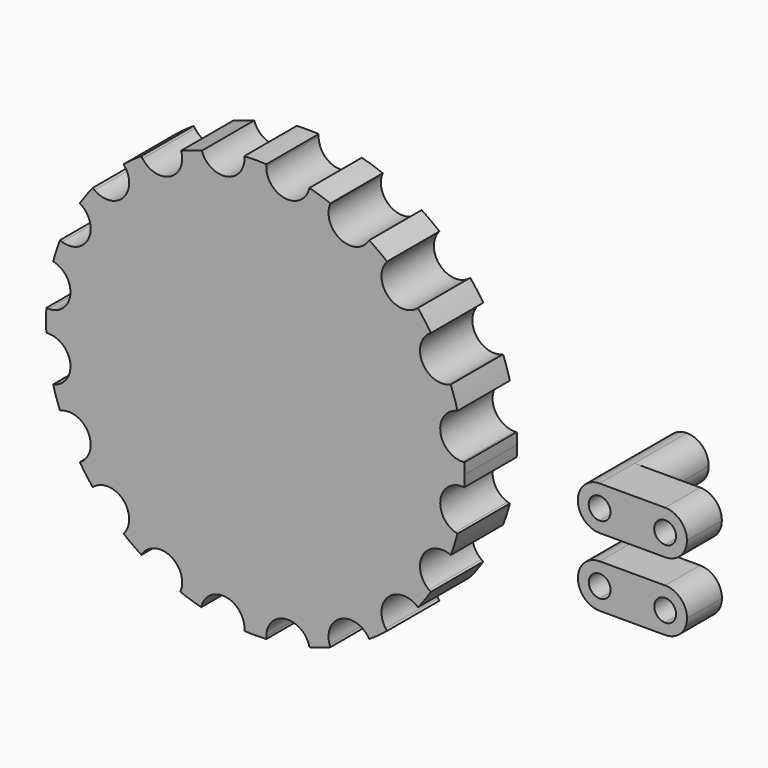
from build123d import *

# Parameters (mm, degrees)
F1_DEPTH = 15
F2_DEPTH = 10
F3_DEPTH = 15
F4_DEPTH = 10


with BuildPart() as f1:
    # F0 (on Front) → F1 (new body)
    with BuildSketch(Plane.XZ):
        with BuildLine():
            Line((47.3531363601, -2.5), (47.3531363601, 2.5))
            ThreePointArc((47.3531363601, 2.5), (42.4146946571, 6.7178276748), (45.8080513882, 12.2552825815))
            Line((45.8080513882, 12.2552825815), (44.2629664163, 17.010565163))
            ThreePointArc((44.2629664163, 17.010565163), (38.2628488235, 19.4958952457), (39.778955183, 25.8109327163))
            Line((39.778955183, 25.8109327163), (36.8400289215, 29.8560176882))
            ThreePointArc((36.8400289215, 29.8560176882), (30.3655687541, 30.3655687541), (29.8560176882, 36.8400289215))
            Line((29.8560176882, 36.8400289215), (25.8109327163, 39.778955183))
            ThreePointArc((25.8109327163, 39.778955183), (19.4958952457, 38.2628488235), (17.010565163, 44.2629664163))
            Line((17.010565163, 44.2629664163), (12.2552825815, 45.8080513882))
            ThreePointArc((12.2552825815, 45.8080513882), (6.7178276748, 42.4146946571), (2.5, 47.3531363601))
            Line((2.5, 47.3531363601), (-2.5, 47.3531363601))
            ThreePointArc((-2.5, 47.3531363601), (-6.7178276748, 42.4146946571), (-12.2552825815, 45.8080513882))
            Line((-12.2552825815, 45.8080513882), (-17.010565163, 44.2629664163))
            ThreePointArc((-17.010565163, 44.2629664163), (-16.8274060415, 43.5000537696), (-16.7658477444, 42.7178814444))
            ThreePointArc((-16.7658477444, 42.7178814444), (-20.2207627726, 37.962598863), (-25.8109327163, 39.778955183))
            Line((-25.8109327163, 39.778955183), (-29.8560176882, 36.8400289215))
            ThreePointArc((-29.8560176882, 36.8400289215), (-29.1458200786, 35.4461876319), (-28.9011026601, 33.9011026601))
            ThreePointArc((-28.9011026601, 33.9011026601), (-31.6311501614, 29.4460700391), (-36.8400289215, 29.8560176882))
            Line((-36.8400289215, 29.8560176882), (-39.778955183, 25.8109327163))
            ThreePointArc((-39.778955183, 25.8109327163), (-38.2628488235, 24.0358002431), (-37.7178814444, 21.7658477444))
            ThreePointArc((-37.7178814444, 21.7658477444), (-39.778955183, 17.7207627726), (-44.2629664163, 17.010565163))
            Line((-44.2629664163, 17.010565163), (-45.8080513882, 12.2552825815))
            ThreePointArc((-45.8080513882, 12.2552825815), (-43.3080513882, 10.4389262615), (-42.3531363601, 7.5))
            ThreePointArc((-42.3531363601, 7.5), (-43.8176024541, 3.9644660941), (-47.3531363601, 2.5))
            Line((-47.3531363601, 2.5), (-47.3531363601, -2.5))
            ThreePointArc((-47.3531363601, -2.5), (-43.8176024541, -3.9644660941), (-42.3531363601, -7.5))
            ThreePointArc((-42.3531363601, -7.5), (-43.3080513882, -10.4389262615), (-45.8080513882, -12.2552825815))
            Line((-45.8080513882, -12.2552825815), (-44.2629664163, -17.010565163))
            ThreePointArc((-44.2629664163, -17.010565163), (-39.778955183, -17.7207627726), (-37.7178814444, -21.7658477444))
            ThreePointArc((-37.7178814444, -21.7658477444), (-38.2628488235, -24.0358002431), (-39.778955183, -25.8109327163))
            Line((-39.778955183, -25.8109327163), (-36.8400289215, -29.8560176882))
            ThreePointArc((-36.8400289215, -29.8560176882), (-31.6311501614, -29.4460700391), (-28.9011026601, -33.9011026601))
            ThreePointArc((-28.9011026601, -33.9011026601), (-29.1458200786, -35.4461876319), (-29.8560176882, -36.8400289215))
            Line((-29.8560176882, -36.8400289215), (-25.8109327163, -39.778955183))
            ThreePointArc((-25.8109327163, -39.778955183), (-20.2207627726, -37.962598863), (-16.7658477444, -42.7178814444))
            ThreePointArc((-16.7658477444, -42.7178814444), (-16.8274060415, -43.5000537696), (-17.010565163, -44.2629664163))
            Line((-17.010565163, -44.2629664163), (-12.2552825815, -45.8080513882))
            ThreePointArc((-12.2552825815, -45.8080513882), (-6.7178276748, -42.4146946571), (-2.5, -47.3531363601))
            Line((-2.5, -47.3531363601), (2.5, -47.3531363601))
            ThreePointArc((2.5, -47.3531363601), (6.7178276748, -42.4146946571), (12.2552825815, -45.8080513882))
            Line((12.2552825815, -45.8080513882), (17.010565163, -44.2629664163))
            ThreePointArc((17.010565163, -44.2629664163), (19.4958952457, -38.2628488235), (25.8109327163, -39.778955183))
            Line((25.8109327163, -39.778955183), (29.8560176882, -36.8400289215))
            ThreePointArc((29.8560176882, -36.8400289215), (30.3655687541, -30.3655687541), (36.8400289215, -29.8560176882))
            Line((36.8400289215, -29.8560176882), (39.778955183, -25.8109327163))
            ThreePointArc((39.778955183, -25.8109327163), (38.2628488235, -19.4958952457), (44.2629664163, -17.010565163))
            Line((44.2629664163, -17.010565163), (45.8080513882, -12.2552825815))
            ThreePointArc((45.8080513882, -12.2552825815), (42.4146946571, -6.7178276748), (47.3531363601, -2.5))
        make_face()
        with BuildLine():
            Line((44.2629664163, 17.010565163), (45.8080513882, 12.2552825815))
            ThreePointArc((45.8080513882, 12.2552825815), (46.0595033261, 12.3297529516), (46.3145139922, 12.3909368813))
            ThreePointArc((46.3145139922, 12.3909368813), (45.5968821856, 14.8153251089), (44.7524388669, 17.1985097785))
            ThreePointArc((44.7524388669, 17.1985097785), (44.5101678926, 17.0981171087), (44.2629664163, 17.010565163))
        make_face()
        with BuildLine():
            ThreePointArc((47.8767304039, 2.5274906458), (47.6152939741, 2.5068773913), (47.3531363601, 2.5))
            Line((47.3531363601, 2.5), (47.3531363601, -2.5))
            ThreePointArc((47.3531363601, -2.5), (47.6152939741, -2.5068773913), (47.8767304039, -2.5274906458))
            ThreePointArc((47.8767304039, -2.5274906458), (47.9267290738, -1.2641848844), (47.9433991612, 0))
            ThreePointArc((47.9433991612, 0), (47.9267290738, 1.2641848844), (47.8767304039, 2.5274906458))
        make_face()
        with BuildLine():
            Line((36.8400289215, 29.8560176882), (39.778955183, 25.8109327163))
            ThreePointArc((39.778955183, 25.8109327163), (39.9950875771, 25.9594611692), (40.2187102588, 26.0964531738))
            ThreePointArc((40.2187102588, 26.0964531738), (38.7870246896, 28.1804229718), (37.247466805, 30.186018945))
            ThreePointArc((37.247466805, 30.186018945), (37.0480764573, 30.0156739939), (36.8400289215, 29.8560176882))
        make_face()
        with BuildLine():
            Line((25.8109327163, 39.778955183), (29.8560176882, 36.8400289215))
            ThreePointArc((29.8560176882, 36.8400289215), (30.0156739939, 37.0480764573), (30.186018945, 37.247466805))
            ThreePointArc((30.186018945, 37.247466805), (28.1804229718, 38.7870246896), (26.0964531738, 40.2187102588))
            ThreePointArc((26.0964531738, 40.2187102588), (25.9594611692, 39.9950875771), (25.8109327163, 39.778955183))
        make_face()
        with BuildLine():
            Line((12.2552825815, 45.8080513882), (17.010565163, 44.2629664163))
            ThreePointArc((17.010565163, 44.2629664163), (17.0981171087, 44.5101678926), (17.1985097785, 44.7524388669))
            ThreePointArc((17.1985097785, 44.7524388669), (14.8153251089, 45.5968821856), (12.3909368813, 46.3145139922))
            ThreePointArc((12.3909368813, 46.3145139922), (12.3297529516, 46.0595033261), (12.2552825815, 45.8080513882))
        make_face()
        with BuildLine():
            Line((-2.5, 47.3531363601), (2.5, 47.3531363601))
            ThreePointArc((2.5, 47.3531363601), (2.5068773913, 47.6152939741), (2.5274906458, 47.8767304039))
            ThreePointArc((2.5274906458, 47.8767304039), (0, 47.9433991612), (-2.5274906458, 47.8767304039))
            ThreePointArc((-2.5274906458, 47.8767304039), (-2.5068773913, 47.6152939741), (-2.5, 47.3531363601))
        make_face()
        with BuildLine():
            ThreePointArc((-25.8109327163, 39.778955183), (-25.9594611692, 39.9950875771), (-26.0964531738, 40.2187102588))
            ThreePointArc((-26.0964531738, 40.2187102588), (-28.1804229718, 38.7870246896), (-30.186018945, 37.247466805))
            ThreePointArc((-30.186018945, 37.247466805), (-30.0156739939, 37.0480764573), (-29.8560176882, 36.8400289215))
            Line((-29.8560176882, 36.8400289215), (-25.8109327163, 39.778955183))
        make_face()
        with BuildLine():
            ThreePointArc((-36.8400289215, 29.8560176882), (-37.0480764573, 30.0156739939), (-37.247466805, 30.186018945))
            ThreePointArc((-37.247466805, 30.186018945), (-38.7870246896, 28.1804229718), (-40.2187102588, 26.0964531738))
            ThreePointArc((-40.2187102588, 26.0964531738), (-39.9950875771, 25.9594611692), (-39.778955183, 25.8109327163))
            Line((-39.778955183, 25.8109327163), (-36.8400289215, 29.8560176882))
        make_face()
        with BuildLine():
            ThreePointArc((-44.2629664163, 17.010565163), (-44.5101678926, 17.0981171087), (-44.7524388669, 17.1985097785))
            ThreePointArc((-44.7524388669, 17.1985097785), (-45.5968821856, 14.8153251089), (-46.3145139922, 12.3909368813))
            ThreePointArc((-46.3145139922, 12.3909368813), (-46.0595033261, 12.3297529516), (-45.8080513882, 12.2552825815))
            Line((-45.8080513882, 12.2552825815), (-44.2629664163, 17.010565163))
        make_face()
        with BuildLine():
            ThreePointArc((-47.3531363601, 2.5), (-47.6152939741, 2.5068773913), (-47.8767304039, 2.5274906458))
            ThreePointArc((-47.8767304039, 2.5274906458), (-47.9433991612, 0), (-47.8767304039, -2.5274906458))
            ThreePointArc((-47.8767304039, -2.5274906458), (-47.6152939741, -2.5068773913), (-47.3531363601, -2.5))
            Line((-47.3531363601, -2.5), (-47.3531363601, 2.5))
        make_face()
        with BuildLine():
            ThreePointArc((-46.3145139922, -12.3909368813), (-45.5968821856, -14.8153251089), (-44.7524388669, -17.1985097785))
            ThreePointArc((-44.7524388669, -17.1985097785), (-44.5101678926, -17.0981171087), (-44.2629664163, -17.010565163))
            Line((-44.2629664163, -17.010565163), (-45.8080513882, -12.2552825815))
            ThreePointArc((-45.8080513882, -12.2552825815), (-46.0595033261, -12.3297529516), (-46.3145139922, -12.3909368813))
        make_face()
        with BuildLine():
            ThreePointArc((-40.2187102588, -26.0964531738), (-38.7870246896, -28.1804229718), (-37.247466805, -30.186018945))
            ThreePointArc((-37.247466805, -30.186018945), (-37.0480764573, -30.0156739939), (-36.8400289215, -29.8560176882))
            Line((-36.8400289215, -29.8560176882), (-39.778955183, -25.8109327163))
            ThreePointArc((-39.778955183, -25.8109327163), (-39.9950875771, -25.9594611692), (-40.2187102588, -26.0964531738))
        make_face()
        with BuildLine():
            ThreePointArc((-30.186018945, -37.247466805), (-28.1804229718, -38.7870246896), (-26.0964531738, -40.2187102588))
            ThreePointArc((-26.0964531738, -40.2187102588), (-25.9594611692, -39.9950875771), (-25.8109327163, -39.778955183))
            Line((-25.8109327163, -39.778955183), (-29.8560176882, -36.8400289215))
            ThreePointArc((-29.8560176882, -36.8400289215), (-30.0156739939, -37.0480764573), (-30.186018945, -37.247466805))
        make_face()
        with BuildLine():
            ThreePointArc((-12.3909368813, -46.3145139922), (-12.3297529516, -46.0595033261), (-12.2552825815, -45.8080513882))
            Line((-12.2552825815, -45.8080513882), (-17.010565163, -44.2629664163))
            ThreePointArc((-17.010565163, -44.2629664163), (-17.0981171087, -44.5101678926), (-17.1985097785, -44.7524388669))
            ThreePointArc((-17.1985097785, -44.7524388669), (-14.8153251089, -45.5968821856), (-12.3909368813, -46.3145139922))
        make_face()
        with BuildLine():
            ThreePointArc((2.5274906458, -47.8767304039), (2.5068773913, -47.6152939741), (2.5, -47.3531363601))
            Line((2.5, -47.3531363601), (-2.5, -47.3531363601))
            ThreePointArc((-2.5, -47.3531363601), (-2.5068773913, -47.6152939741), (-2.5274906458, -47.8767304039))
            ThreePointArc((-2.5274906458, -47.8767304039), (0, -47.9433991612), (2.5274906458, -47.8767304039))
        make_face()
        with BuildLine():
            ThreePointArc((17.1985097785, -44.7524388669), (17.0981171087, -44.5101678926), (17.010565163, -44.2629664163))
            Line((17.010565163, -44.2629664163), (12.2552825815, -45.8080513882))
            ThreePointArc((12.2552825815, -45.8080513882), (12.3297529516, -46.0595033261), (12.3909368813, -46.3145139922))
            ThreePointArc((12.3909368813, -46.3145139922), (14.8153251089, -45.5968821856), (17.1985097785, -44.7524388669))
        make_face()
        with BuildLine():
            ThreePointArc((30.186018945, -37.247466805), (30.0156739939, -37.0480764573), (29.8560176882, -36.8400289215))
            Line((29.8560176882, -36.8400289215), (25.8109327163, -39.778955183))
            ThreePointArc((25.8109327163, -39.778955183), (25.9594611692, -39.9950875771), (26.0964531738, -40.2187102588))
            ThreePointArc((26.0964531738, -40.2187102588), (28.1804229718, -38.7870246896), (30.186018945, -37.247466805))
        make_face()
        with BuildLine():
            ThreePointArc((40.2187102588, -26.0964531738), (39.9950875771, -25.9594611692), (39.778955183, -25.8109327163))
            Line((39.778955183, -25.8109327163), (36.8400289215, -29.8560176882))
            ThreePointArc((36.8400289215, -29.8560176882), (37.0480764573, -30.0156739939), (37.247466805, -30.186018945))
            ThreePointArc((37.247466805, -30.186018945), (38.7870246896, -28.1804229718), (40.2187102588, -26.0964531738))
        make_face()
        with BuildLine():
            ThreePointArc((46.3145139922, -12.3909368813), (46.0595033261, -12.3297529516), (45.8080513882, -12.2552825815))
            Line((45.8080513882, -12.2552825815), (44.2629664163, -17.010565163))
            ThreePointArc((44.2629664163, -17.010565163), (44.5101678926, -17.0981171087), (44.7524388669, -17.1985097785))
            ThreePointArc((44.7524388669, -17.1985097785), (45.5968821856, -14.8153251089), (46.3145139922, -12.3909368813))
        make_face()
    extrude(amount=F1_DEPTH)


with BuildPart() as f2:
    # F0 (on Front) → F2 (new body)
    with BuildSketch(Plane.XZ):
        with BuildLine():
            ThreePointArc((74.8708024621, 5), (78.406336368, 3.5355339059), (79.8708024621, 0))
            ThreePointArc((79.8708024621, 0), (78.406336368, -3.5355339059), (74.8708024621, -5))
            Line((74.8708024621, -5), (89.8708024621, -5))
            ThreePointArc((89.8708024621, -5), (84.8708024621, 0), (89.8708024621, 5))
            Line((89.8708024621, 5), (74.8708024621, 5))
        make_face()
        with BuildLine():
            ThreePointArc((74.8708024621, -5), (78.406336368, -3.5355339059), (79.8708024621, 0))
            ThreePointArc((79.8708024621, 0), (78.406336368, 3.5355339059), (74.8708024621, 5))
            Line((74.8708024621, 5), (74.8708024621, 2.5))
            ThreePointArc((74.8708024621, 2.5), (76.6385694151, 1.767766953), (77.3708024621, 0))
            ThreePointArc((77.3708024621, 0), (76.6385694151, -1.767766953), (74.8708024621, -2.5))
            Line((74.8708024621, -2.5), (74.8708024621, -5))
        make_face()
        with BuildLine():
            Line((74.8708024621, 2.5), (74.8708024621, 5))
            ThreePointArc((74.8708024621, 5), (69.8708024621, 0), (74.8708024621, -5))
            Line((74.8708024621, -5), (74.8708024621, -2.5))
            ThreePointArc((74.8708024621, -2.5), (72.3708024621, 0), (74.8708024621, 2.5))
        make_face()
        with BuildLine():
            Line((89.8708024621, 2.5), (89.8708024621, 5))
            ThreePointArc((89.8708024621, 5), (84.8708024621, 0), (89.8708024621, -5))
            Line((89.8708024621, -5), (89.8708024621, -2.5))
            ThreePointArc((89.8708024621, -2.5), (87.3708024621, 0), (89.8708024621, 2.5))
        make_face()
        with BuildLine():
            ThreePointArc((94.8708024621, 0), (93.406336368, 3.5355339059), (89.8708024621, 5))
            Line((89.8708024621, 5), (89.8708024621, 2.5))
            ThreePointArc((89.8708024621, 2.5), (91.6385694151, 1.767766953), (92.3708024621, 0))
            ThreePointArc((92.3708024621, 0), (91.6385694151, -1.767766953), (89.8708024621, -2.5))
            Line((89.8708024621, -2.5), (89.8708024621, -5))
            ThreePointArc((89.8708024621, -5), (93.406336368, -3.5355339059), (94.8708024621, 0))
        make_face()
    extrude(amount=F2_DEPTH)

    # F0 (on Front) → F3 (join)
    with BuildSketch(Plane.XZ):
        with BuildLine():
            Line((74.8708024621, 2.5), (74.8708024621, 5))
            ThreePointArc((74.8708024621, 5), (69.8708024621, 0), (74.8708024621, -5))
            Line((74.8708024621, -5), (74.8708024621, -2.5))
            ThreePointArc((74.8708024621, -2.5), (72.3708024621, 0), (74.8708024621, 2.5))
        make_face()
        with BuildLine():
            ThreePointArc((74.8708024621, -5), (78.406336368, -3.5355339059), (79.8708024621, 0))
            ThreePointArc((79.8708024621, 0), (78.406336368, 3.5355339059), (74.8708024621, 5))
            Line((74.8708024621, 5), (74.8708024621, 2.5))
            ThreePointArc((74.8708024621, 2.5), (76.6385694151, 1.767766953), (77.3708024621, 0))
            ThreePointArc((77.3708024621, 0), (76.6385694151, -1.767766953), (74.8708024621, -2.5))
            Line((74.8708024621, -2.5), (74.8708024621, -5))
        make_face()
    extrude(amount=-F3_DEPTH)


with BuildPart() as f4:
    # F0 (on Front) → F4 (new body)
    with BuildSketch(Plane.XZ):
        with BuildLine():
            Line((89.8868063092, -10.6893767416), (74.8868063092, -10.6893767416))
            ThreePointArc((74.8868063092, -10.6893767416), (78.4223402152, -12.1538428357), (79.8868063092, -15.6893767416))
            ThreePointArc((79.8868063092, -15.6893767416), (78.4223402152, -19.2249106476), (74.8868063092, -20.6893767416))
            Line((74.8868063092, -20.6893767416), (89.8868063092, -20.6893767416))
            ThreePointArc((89.8868063092, -20.6893767416), (84.8868063092, -15.6893767416), (89.8868063092, -10.6893767416))
        make_face()
        with BuildLine():
            ThreePointArc((74.8868063092, -13.1893767416), (76.6545732622, -13.9216097887), (77.3868063092, -15.6893767416))
            ThreePointArc((77.3868063092, -15.6893767416), (76.6545732622, -17.4571436946), (74.8868063092, -18.1893767416))
            Line((74.8868063092, -18.1893767416), (74.8868063092, -20.6893767416))
            ThreePointArc((74.8868063092, -20.6893767416), (78.4223402152, -19.2249106476), (79.8868063092, -15.6893767416))
            ThreePointArc((79.8868063092, -15.6893767416), (78.4223402152, -12.1538428357), (74.8868063092, -10.6893767416))
            Line((74.8868063092, -10.6893767416), (74.8868063092, -13.1893767416))
        make_face()
        with BuildLine():
            ThreePointArc((74.8868063092, -18.1893767416), (72.3868063092, -15.6893767416), (74.8868063092, -13.1893767416))
            Line((74.8868063092, -13.1893767416), (74.8868063092, -10.6893767416))
            ThreePointArc((74.8868063092, -10.6893767416), (69.8868063092, -15.6893767416), (74.8868063092, -20.6893767416))
            Line((74.8868063092, -20.6893767416), (74.8868063092, -18.1893767416))
        make_face()
        with BuildLine():
            Line((89.8868063092, -13.1893767416), (89.8868063092, -10.6893767416))
            ThreePointArc((89.8868063092, -10.6893767416), (84.8868063092, -15.6893767416), (89.8868063092, -20.6893767416))
            Line((89.8868063092, -20.6893767416), (89.8868063092, -18.1893767416))
            ThreePointArc((89.8868063092, -18.1893767416), (87.3868063092, -15.6893767416), (89.8868063092, -13.1893767416))
        make_face()
        with BuildLine():
            ThreePointArc((94.8868063092, -15.6893767416), (93.4223402152, -12.1538428357), (89.8868063092, -10.6893767416))
            Line((89.8868063092, -10.6893767416), (89.8868063092, -13.1893767416))
            ThreePointArc((89.8868063092, -13.1893767416), (91.6545732622, -13.9216097887), (92.3868063092, -15.6893767416))
            ThreePointArc((92.3868063092, -15.6893767416), (91.6545732622, -17.4571436946), (89.8868063092, -18.1893767416))
            Line((89.8868063092, -18.1893767416), (89.8868063092, -20.6893767416))
            ThreePointArc((89.8868063092, -20.6893767416), (93.4223402152, -19.2249106476), (94.8868063092, -15.6893767416))
        make_face()
    extrude(amount=F4_DEPTH)


solid = Compound([f1.part, f2.part, f4.part])
